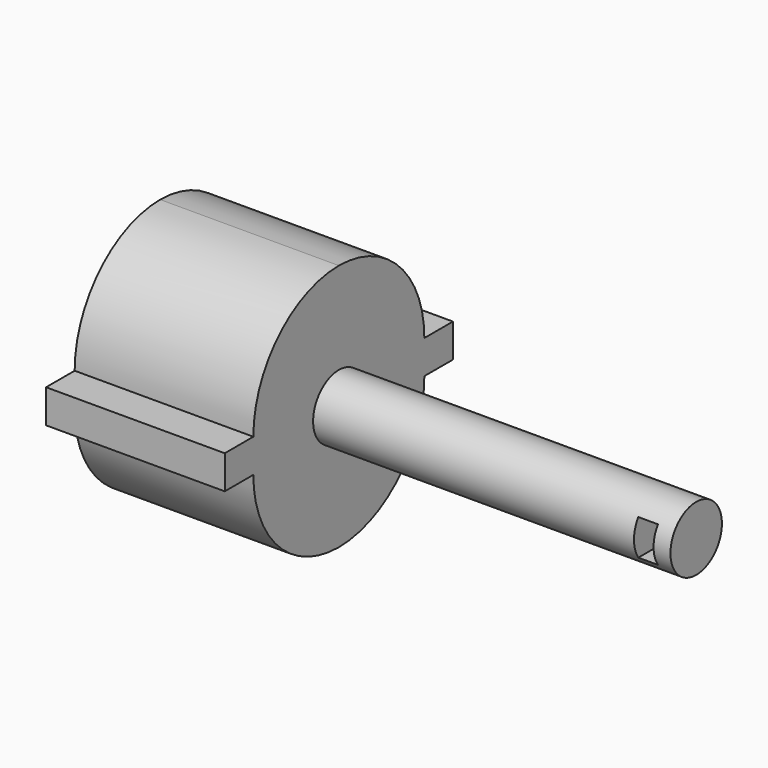
from build123d import *

# Parameters (mm, degrees)
F0_W        = 29.9085080624
F0_H        = 34.6928238869
F1_DEPTH    = 25
F2_R        = 4.5021693383
F3_DEPTH    = 50
F4_T1_DEPTH = 100
F5_DEPTH    = 5
F6_DEPTH    = 5
F8_DEPTH    = 2.5


# Not quite as in the source:
# - a fillet or chamfer that OpenCascade refuses, or shapes differently, is made with other operations: its cross-section is extruded or revolved along the edge and cut away or added


with BuildPart() as f1:
    # F0 (on Right) → F1 (new body)
    with BuildSketch(Plane.YZ):
        Rectangle(F0_W, F0_H)
    extrude(amount=-F1_DEPTH)

    # F2 (on Right) → F3 (join)
    with BuildSketch(Plane.YZ):
        Circle(F2_R)
    extrude(amount=F3_DEPTH)

    # F4: fillet of radius 15 on 4 edges, made by hand

    # F4_s2 → F4_t1 (cut)
    with BuildSketch(Plane.YZ.offset(-62.5)):
        with BuildLine():
            ThreePointArc((0.0457459688, 17.3464119434), (-10.560855749, 12.9530136612), (-14.9542540312, 2.3464119434))
            Line((-14.9542540312, 2.3464119434), (-14.9542540312, 17.3464119434))
            Line((-14.9542540312, 17.3464119434), (0.0457459688, 17.3464119434))
        make_face()
        with BuildLine():
            ThreePointArc((14.9542540312, -2.3464119434), (10.560855749, -12.9530136612), (-0.0457459688, -17.3464119434))
            Line((-0.0457459688, -17.3464119434), (14.9542540312, -17.3464119434))
            Line((14.9542540312, -17.3464119434), (14.9542540312, -2.3464119434))
        make_face()
        with BuildLine():
            ThreePointArc((14.9542540312, 2.3464119434), (10.560855749, 12.9530136612), (-0.0457459688, 17.3464119434))
            Line((-0.0457459688, 17.3464119434), (14.9542540312, 17.3464119434))
            Line((14.9542540312, 17.3464119434), (14.9542540312, 2.3464119434))
        make_face()
        with BuildLine():
            ThreePointArc((0.0457459688, -17.3464119434), (-10.560855749, -12.9530136612), (-14.9542540312, -2.3464119434))
            Line((-14.9542540312, -2.3464119434), (-14.9542540312, -17.3464119434))
            Line((-14.9542540312, -17.3464119434), (0.0457459688, -17.3464119434))
        make_face()
    extrude(amount=F4_T1_DEPTH, mode=Mode.SUBTRACT)

    # F5 (add): a face of the model
    f5_faces = [f1.faces().sort_by_distance(p)[0] for p in [
        (-12.5, 14.9542540312, 0),
    ]]
    extrude(f5_faces, amount=F5_DEPTH)

    # F6 (add): a face of the model
    f6_faces = [f1.faces().sort_by_distance(p)[0] for p in [
        (-12.5, -14.9542540312, 0),
    ]]
    extrude(f6_faces, amount=F6_DEPTH)

    # F7 (on Top) → F8 (cut, symmetric)
    with BuildSketch(Plane.XY):
        Polygon((44.8985174298, 7.189091295), (44.8985174298, -8.9538004249), (47.6411059499, -8.9538004249), (47.6411059499, 6.886465475), align=None)
    extrude(amount=F8_DEPTH, both=True, mode=Mode.SUBTRACT)


solid = f1.part
